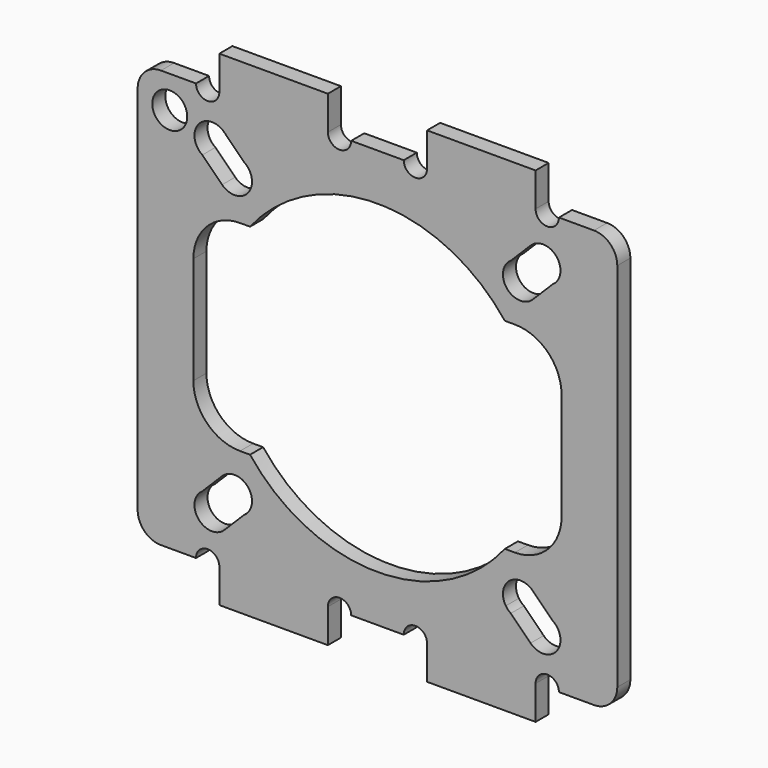
from build123d import *

# Parameters (mm, degrees)
F0_R     = 1.5
F0_W     = 9.3
F0_H     = 2.9
F1_DEPTH = 1.4
F2_R     = 4
F3_DEPTH = 2
F4_R     = 2


# Not quite as in the source:
# - a pattern or mirror of a feature is missing from the dataset's text; its kind, count and spacing are read off the source's solid
# - a feature names something its author has since deleted; it is built from what else it names


with BuildPart() as f1:
    # F0 (on Front) → F1 (new body)
    with BuildSketch(Plane.XZ):
        with BuildLine():
            Line((15.55, -17.9), (20.55, -17.9))
            Line((20.55, -17.9), (20.55, 17.9))
            Line((20.55, 17.9), (15.55, 17.9))
            ThreePointArc((15.55, 17.9), (14.55, 16.9), (13.55, 17.9))
            Line((13.55, 17.9), (4.25, 17.9))
            ThreePointArc((4.25, 17.9), (3.25, 16.9), (2.25, 17.9))
            Line((2.25, 17.9), (-2.25, 17.9))
            ThreePointArc((-2.25, 17.9), (-3.25, 16.9), (-4.25, 17.9))
            Line((-4.25, 17.9), (-13.55, 17.9))
            ThreePointArc((-13.55, 17.9), (-14.55, 16.9), (-15.55, 17.9))
            Line((-15.55, 17.9), (-20.55, 17.9))
            Line((-20.55, 17.9), (-20.55, -17.9))
            Line((-20.55, -17.9), (-15.55, -17.9))
            ThreePointArc((-15.55, -17.9), (-14.55, -16.9), (-13.55, -17.9))
            Line((-13.55, -17.9), (-4.25, -17.9))
            ThreePointArc((-4.25, -17.9), (-3.25, -16.9), (-2.25, -17.9))
            Line((-2.25, -17.9), (2.25, -17.9))
            ThreePointArc((2.25, -17.9), (3.25, -16.9), (4.25, -17.9))
            Line((4.25, -17.9), (13.55, -17.9))
            ThreePointArc((13.55, -17.9), (14.55, -16.9), (15.55, -17.9))
        make_face()
        with BuildLine():
            ThreePointArc((-13.1202274148, -14.9978997242), (-15.343659863, -14.8848474001), (-15.0056689733, -12.6843486297))
            Line((-15.0056689733, -12.6843486297), (-13.3106601718, -10.9893398282))
            ThreePointArc((-13.3106601718, -10.9893398282), (-11.6759748515, -10.6641807012), (-10.75, -12.05))
            ThreePointArc((-10.75, -12.05), (-10.8131046691, -12.4805018095), (-10.9971090773, -12.8747813867))
            ThreePointArc((-10.9971090773, -12.8747813867), (-11.1893398282, -13.1106601718), (-11.4252186133, -13.3028909227))
            Line((-11.4252186133, -13.3028909227), (-13.1202274148, -14.9978997242))
        make_face(mode=Mode.SUBTRACT)
        with BuildLine():
            Line((13.3106601718, -10.9893398282), (15.0056689733, -12.6843486297))
            ThreePointArc((15.0056689733, -12.6843486297), (15.5013367677, -13.2256118689), (15.6808875866, -13.9372395524))
            ThreePointArc((15.6808875866, -13.9372395524), (14.7549127351, -15.3230588512), (13.1202274148, -14.9978997242))
            Line((13.1202274148, -14.9978997242), (11.4252186133, -13.3028909227))
            ThreePointArc((11.4252186133, -13.3028909227), (11.1893398282, -13.1106601718), (10.9971090773, -12.8747813867))
            ThreePointArc((10.9971090773, -12.8747813867), (11.3023921523, -10.8872277235), (13.3106601718, -10.9893398282))
        make_face(mode=Mode.SUBTRACT)
        with Locations((-17.8, 15.15)):
            Circle(F0_R, mode=Mode.SUBTRACT)
        with BuildLine():
            ThreePointArc((-15.0056689733, 12.6843486297), (-15.343659863, 14.8848474001), (-13.1202274148, 14.9978997242))
            Line((-13.1202274148, 14.9978997242), (-11.4252186133, 13.3028909227))
            ThreePointArc((-11.4252186133, 13.3028909227), (-11.1893398282, 13.1106601718), (-10.9971090773, 12.8747813867))
            ThreePointArc((-10.9971090773, 12.8747813867), (-10.8131046691, 12.4805018095), (-10.75, 12.05))
            ThreePointArc((-10.75, 12.05), (-11.6759748515, 10.6641807012), (-13.3106601718, 10.9893398282))
            Line((-13.3106601718, 10.9893398282), (-15.0056689733, 12.6843486297))
        make_face(mode=Mode.SUBTRACT)
        with BuildLine():
            ThreePointArc((-10.9201648339, 8.6), (0, 13.9), (10.9201648339, 8.6))
            Line((10.9201648339, 8.6), (15.775, 8.6))
            Line((15.775, 8.6), (15.775, -8.6))
            Line((15.775, -8.6), (10.9201648339, -8.6))
            ThreePointArc((10.9201648339, -8.6), (0, -13.9), (-10.9201648339, -8.6))
            Line((-10.9201648339, -8.6), (-15.775, -8.6))
            Line((-15.775, -8.6), (-15.775, 8.6))
            Line((-15.775, 8.6), (-10.9201648339, 8.6))
        make_face(mode=Mode.SUBTRACT)
        with BuildLine():
            ThreePointArc((13.1202274148, 14.9978997242), (14.7549127351, 15.3230588512), (15.6808875866, 13.9372395524))
            ThreePointArc((15.6808875866, 13.9372395524), (15.5013367677, 13.2256118689), (15.0056689733, 12.6843486297))
            Line((15.0056689733, 12.6843486297), (13.3106601718, 10.9893398282))
            ThreePointArc((13.3106601718, 10.9893398282), (11.3023921523, 10.8872277235), (10.9971090773, 12.8747813867))
            ThreePointArc((10.9971090773, 12.8747813867), (11.1893398282, 13.1106601718), (11.4252186133, 13.3028909227))
            Line((11.4252186133, 13.3028909227), (13.1202274148, 14.9978997242))
        make_face(mode=Mode.SUBTRACT)
        with Locations((-8.9, -19.35)):
            Rectangle(F0_W, F0_H)
        with Locations((8.9, -19.35)):
            Rectangle(F0_W, F0_H)
        with Locations((8.9, 19.35)):
            Rectangle(F0_W, F0_H)
    extrude(amount=F1_DEPTH)

    # F1_copies: F1 across plane


with BuildPart() as f1_1:
    add(f1.part)
    add(f1.part.mirror(Plane.XY))

    # F2
    f2_edges = [f1_1.edges().sort_by_distance(p)[0] for p in [
        (-15.775, -0.7, 8.6),
        (-15.775, -0.7, -8.6),
        (15.775, -0.7, 8.6),
        (15.775, -0.7, -8.6),
    ]]
    fillet(f2_edges, radius=F2_R)

    # F0 (on Front) → F3 (cut)
    with BuildSketch(Plane.XZ):
        with BuildLine():
            ThreePointArc((-4.25, 17.9), (-3.25, 16.9), (-2.25, 17.9))
            Line((-2.25, 17.9), (-4.25, 17.9))
        make_face()
        with BuildLine():
            Line((-4.25, 17.9), (-2.25, 17.9))
            ThreePointArc((-2.25, 17.9), (-3.25, 18.9), (-4.25, 17.9))
        make_face()
        with Locations((-17.8, 15.15)):
            Circle(F0_R)
    extrude(amount=F3_DEPTH, mode=Mode.SUBTRACT)

    # F4
    f4_edges = [f1_1.edges().sort_by_distance(p)[0] for p in [
        (-20.55, -0.7, 17.9),
        (20.55, -0.7, 17.9),
        (20.55, -0.7, -17.9),
        (-20.55, -0.7, -17.9),
    ]]
    fillet(f4_edges, radius=F4_R)


solid = f1_1.part
